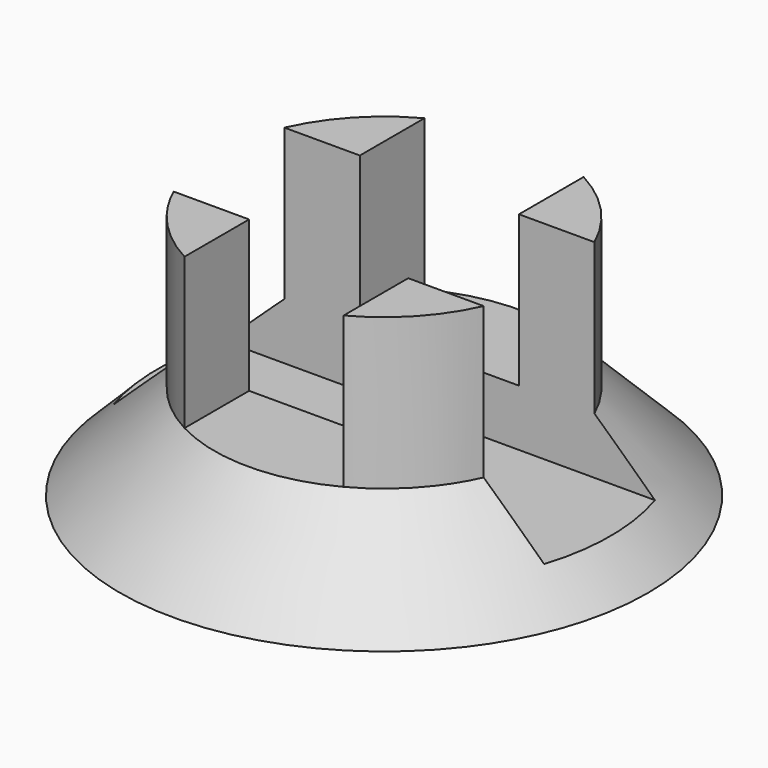
from build123d import *

# Parameters (mm, degrees)
F1_DEPTH    = 5.08
F2_SIZE     = 5.07999
F3_DEPTH    = 12.7
F4_DEPTH    = 12.7
F5_T2_ANGLE = 254.9699407606
F5_T4_ANGLE = 254.9699407606
F8_DEPTH    = 20.32
F9_DEPTH    = 20.32


# Not quite as in the source:
# - a fillet or chamfer that OpenCascade refuses, or shapes differently, is made with other operations: its cross-section is extruded or revolved along the edge and cut away or added
# - a fillet or chamfer is up to 0.001 mm smaller than in the source, because OpenCascade refuses the exact size


with BuildPart() as f1:
    # F0 (on Top) → F1 (new body)
    with BuildSketch(Plane.XY):
        with BuildLine():
            ThreePointArc((34.3164340333, -9.3218), (35.2477374751, -4.7021912858), (35.56, 0))
            ThreePointArc((35.56, 0), (35.2477374751, 4.7021912858), (34.3164340333, 9.3218))
            Line((34.3164340333, 9.3218), (-34.3164340333, 9.3218))
            ThreePointArc((-34.3164340333, 9.3218), (-35.56, 0), (-34.3164340333, -9.3218))
            Line((-34.3164340333, -9.3218), (34.3164340333, -9.3218))
        make_face()
    extrude(amount=F1_DEPTH)

    # F2 (size 5.08 in the source; OpenCascade refuses exactly that, so slightly less here)
    f2_edges = [f1.edges().sort_by_distance(p)[0] for p in [
        (35.56, 0, 5.08),
        (-35.56, 0, 5.08),
    ]]
    chamfer(f2_edges, length=F2_SIZE)

    # F0 (on Top) → F3 (join)
    with BuildSketch(Plane.XY):
        with BuildLine():
            ThreePointArc((-34.3164340333, -9.3218), (0, -35.56), (34.3164340333, -9.3218))
            Line((34.3164340333, -9.3218), (-34.3164340333, -9.3218))
        make_face()
    extrude(amount=F3_DEPTH)

    # F0 (on Top) → F4 (join)
    with BuildSketch(Plane.XY):
        with BuildLine():
            Line((-34.3164340333, 9.3218), (34.3164340333, 9.3218))
            ThreePointArc((34.3164340333, 9.3218), (0, 35.56), (-34.3164340333, 9.3218))
        make_face()
    extrude(amount=F4_DEPTH)

    # F5: chamfer of 12.7 on 2 edges, made by hand

    # F5_s1 → F5_t2 (revolve, cut)
    with BuildSketch(Plane(origin=(0, 0, 0), x_dir=(0, 0, 1), z_dir=(-0.6085532985, -0.7935130011, 0))):
        Polygon((0, -35.56), (12.7, -22.86), (12.7, -35.56), align=None)
    revolve(axis=Axis((0, 0, 12.7), (0, 0, 1)), revolution_arc=F5_T2_ANGLE, mode=Mode.SUBTRACT)

    # F5_s3 → F5_t4 (revolve, cut)
    with BuildSketch(Plane(origin=(0, 0, 0), x_dir=(0, 0, 1), z_dir=(0.6085532985, 0.7935130011, 0))):
        Polygon((0, -35.56), (12.7, -22.86), (12.7, -35.56), align=None)
    revolve(axis=Axis((0, 0, 12.7), (0, 0, 1)), revolution_arc=F5_T4_ANGLE, mode=Mode.SUBTRACT)

    # F6 (on face) → F8 (join)
    with BuildSketch(Plane.XY.offset(12.7)):
        with BuildLine():
            Line((-10.7130363091, -20.1943173452), (-10.7130363091, -9.3218))
            Line((-10.7130363091, -9.3218), (-20.8730363091, -9.3218))
            ThreePointArc((-20.8730363091, -9.3218), (-19.6408996947, -11.6967798638), (-18.1397072045, -13.911528404))
            ThreePointArc((-18.1397072045, -13.911528404), (-14.7644356914, -17.4525367416), (-10.7130363091, -20.1943173452))
        make_face()
        with BuildLine():
            ThreePointArc((10.7130363091, -20.1943173452), (16.7024819777, -15.6079049134), (20.8730363091, -9.3218))
            Line((20.8730363091, -9.3218), (10.7130363091, -9.3218))
            Line((10.7130363091, -9.3218), (10.7130363091, -20.1943173452))
        make_face()
    extrude(amount=F8_DEPTH)

    # F7 (on face) → F9 (join)
    with BuildSketch(Plane.XY.offset(12.7)):
        with BuildLine():
            Line((10.7130363091, 9.3218), (20.8730363091, 9.3218))
            ThreePointArc((20.8730363091, 9.3218), (16.7024819777, 15.6079049134), (10.7130363091, 20.1943173452))
            Line((10.7130363091, 20.1943173452), (10.7130363091, 9.3218))
        make_face()
        with BuildLine():
            Line((-20.8730363091, 9.3218), (-10.7130363091, 9.3218))
            Line((-10.7130363091, 9.3218), (-10.7130363091, 20.1943173452))
            ThreePointArc((-10.7130363091, 20.1943173452), (-16.7024819777, 15.6079049134), (-20.8730363091, 9.3218))
        make_face()
    extrude(amount=F9_DEPTH)


solid = f1.part
